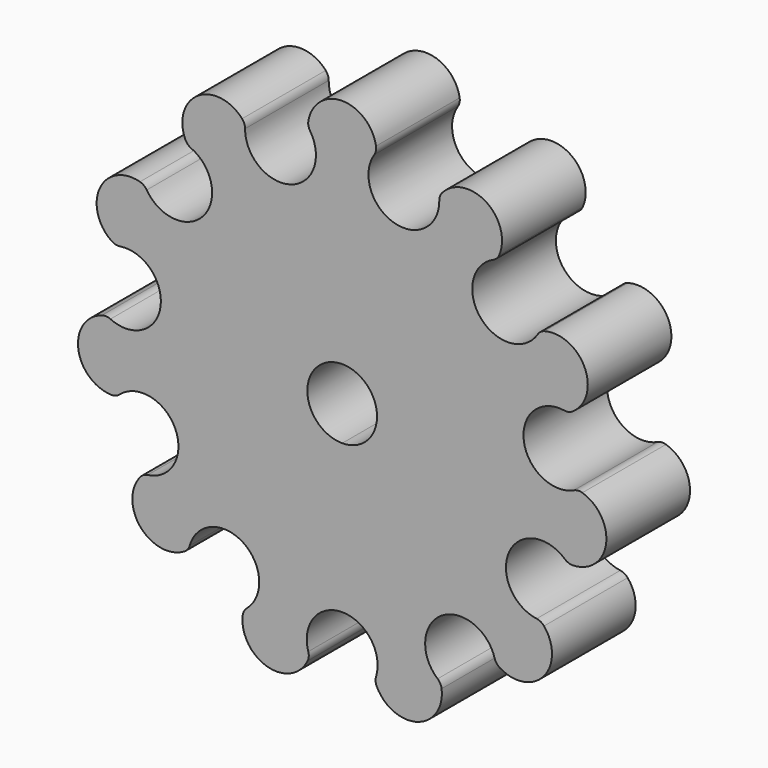
from build123d import *

# Parameters (mm, degrees)
F1_DEPTH = 9
F3_DEPTH = 25
F4_R     = 1


# Not quite as in the source:
# - a feature names something its author has since deleted; it is built from what else it names


with BuildPart() as f1:
    # F0 (on Front) → F1 (new body)
    with BuildSketch(Plane.XZ):
        with BuildLine():
            ThreePointArc((19.6162560617, 5.6676338172), (21.0365592627, 7.3533200275), (20.9215180503, 9.5545843692))
            ThreePointArc((20.9215180503, 9.5545843692), (19.3332494727, 11.0830336302), (17.1292022042, 11.1135271735))
            ThreePointArc((17.1292022042, 11.1135271735), (16.9792927626, 11.0241147009), (16.8692526077, 10.8886208073))
            ThreePointArc((16.8692526077, 10.8886208073), (14.5941945388, 9.3646392479), (12.0291450919, 10.3232477941))
            ThreePointArc((12.0291450919, 10.3232477941), (14.4190139917, 6.5849686535), (15.6791980607, 2.3307777312))
            ThreePointArc((15.6791980607, 2.3307777312), (16.6344691132, 4.8970674002), (19.2760557108, 5.6184589003))
            ThreePointArc((19.2760557108, 5.6184589003), (19.4505144763, 5.6128928995), (19.6162560617, 5.6676338172))
        make_face()
        with BuildLine():
            ThreePointArc((19.5663988928, -5.8374317411), (21.6725847499, -5.1872161444), (22.7658992762, -3.2731987637))
            ThreePointArc((22.7658992762, -3.2731987637), (22.2561047811, -1.1287026022), (20.4184282847, 0.0885481149))
            ThreePointArc((20.4184282847, 0.0885481149), (20.2439764052, 0.0943767195), (20.0781512067, 0.0398842021))
            ThreePointArc((20.0781512067, 0.0398842021), (17.3403239328, -0.0121814146), (15.7007299317, 2.1810218413))
            ThreePointArc((15.7007299317, 2.1810218413), (15.8137560479, 1.0931131305), (15.8514913071, 0))
            ThreePointArc((15.8514913071, 0), (15.497233491, -3.3324961792), (14.4502943385, -6.5160394559))
            ThreePointArc((14.4502943385, -6.5160394559), (16.6413604307, -4.8735977283), (19.2536181785, -5.6948741179))
            ThreePointArc((19.2536181785, -5.6948741179), (19.397373024, -5.7938760653), (19.5663988928, -5.8374317411))
        make_face()
        with BuildLine():
            ThreePointArc((13.4380905328, 15.3732656841), (13.7215754547, 17.5592266426), (12.4347068413, 19.3488517946))
            ThreePointArc((12.4347068413, 19.3488517946), (10.272226498, 19.7759854418), (8.4015754529, 18.610039879))
            ThreePointArc((8.4015754529, 18.610039879), (8.3238036379, 18.4537741575), (8.3044854982, 18.2802972415))
            ThreePointArc((8.3044854982, 18.2802972415), (7.2145114964, 15.7682531166), (4.5383916793, 15.1879155128))
            ThreePointArc((4.5383916793, 15.1879155128), (8.5699436247, 13.3351356547), (11.9300671826, 10.4375894572))
            ThreePointArc((11.9300671826, 10.4375894572), (11.3462513859, 13.1129482303), (13.1784817531, 15.1479709158))
            ThreePointArc((13.1784817531, 15.1479709158), (13.3282550131, 15.2376080275), (13.4380905328, 15.3732656841))
        make_face()
        with BuildLine():
            ThreePointArc((13.304348325, -15.4891539669), (15.4277177081, -16.0808478428), (17.3822683366, -15.061764421))
            ThreePointArc((17.3822683366, -15.061764421), (18.1128040767, -12.9820837356), (17.2249476546, -10.9645443445))
            ThreePointArc((17.2249476546, -10.9645443445), (17.0813405762, -10.8653252035), (16.9123786629, -10.8215153555))
            ThreePointArc((16.9123786629, -10.8215153555), (14.581022999, -9.385134564), (14.3874439542, -6.6536631357))
            ThreePointArc((14.3874439542, -6.6536631357), (11.9797730605, -10.3805016295), (8.6335242647, -13.294060156))
            ThreePointArc((8.6335242647, -13.294060156), (11.3647373936, -13.0969300134), (13.1182929141, -15.2001248417))
            ThreePointArc((13.1182929141, -15.2001248417), (13.1857026919, -15.3611303169), (13.304348325, -15.4891539669))
        make_face()
        with BuildLine():
            ThreePointArc((2.9934262088, 20.1979943186), (2.0500891812, 22.1902052175), (-3.79913e-05, 23))
            ThreePointArc((-3.79913e-05, 23), (-2.0501581038, 22.190202549), (-2.9934921419, 20.1979964151))
            ThreePointArc((-2.9934921419, 20.1979964151), (-2.9744343287, 20.0244907072), (-2.8968970802, 19.8681084639))
            ThreePointArc((-2.8968970802, 19.8681084639), (-2.4557279708, 17.1655580339), (-4.3932690247, 15.2305273689))
            ThreePointArc((-4.3932690247, 15.2305273689), (-2.32908e-05, 15.8514913071), (4.3932242679, 15.2305402791))
            ThreePointArc((4.3932242679, 15.2305402791), (2.4556790123, 17.1655606489), (2.8968329534, 19.8681091959))
            ThreePointArc((2.8968329534, 19.8681091959), (2.9743687562, 20.0244902705), (2.9934262088, 20.1979943186))
        make_face()
        with BuildLine():
            ThreePointArc((2.818261168, -20.2231792494), (4.2846548782, -21.8689217424), (6.4798805109, -22.0683290841))
            ThreePointArc((6.4798805109, -22.0683290841), (8.2188135394, -20.7137492759), (8.5626678499, -18.5364714463))
            ThreePointArc((8.5626678499, -18.5364714463), (8.4954998052, -18.3753631452), (8.3770453909, -18.2471602488))
            ThreePointArc((8.3770453909, -18.2471602488), (7.1923502876, -15.7783738016), (8.5062461781, -13.3758570797))
            ThreePointArc((8.5062461781, -13.3758570797), (4.4659035231, -15.2093879687), (0.0756712384, -15.8513106879))
            ThreePointArc((0.0756712384, -15.8513106879), (2.4798905335, -17.1620795577), (2.8180023388, -19.8794433272))
            ThreePointArc((2.8180023388, -19.8794433272), (2.7876649209, -20.0513342295), (2.818261168, -20.2231792494))
        make_face()
        with BuildLine():
            ThreePointArc((-8.4016297859, 18.6100024692), (-10.2722859221, 19.7759504243), (-12.4347707621, 19.3488107152))
            ThreePointArc((-12.4347707621, 19.3488107152), (-13.7216319934, 17.5591871352), (-13.4381471327, 15.3732318016))
            ThreePointArc((-13.4381471327, 15.3732318016), (-13.3283104123, 15.2375729436), (-13.1785353042, 15.1479356304))
            ThreePointArc((-13.1785353042, 15.1479356304), (-11.3462911586, 13.1129195615), (-11.9300978548, 10.4375543992))
            ThreePointArc((-11.9300978548, 10.4375543992), (-8.5699828116, 13.3351104708), (-4.5384363109, 15.1879021761))
            ThreePointArc((-4.5384363109, 15.1879021761), (-7.2145540967, 15.7682288475), (-8.3045398409, 18.2802631877))
            ThreePointArc((-8.3045398409, 18.2802631877), (-8.3238585649, 18.453738339), (-8.4016297859, 18.6100024692))
        make_face()
        with BuildLine():
            ThreePointArc((15.7007299317, 2.1810218413), (15.6890197856, 2.2557640279), (15.6791980607, 2.3307777312))
            ThreePointArc((15.6791980607, 2.3307777312), (14.4190139917, 6.5849686535), (12.0291450919, 10.3232477941))
            ThreePointArc((12.0291450919, 10.3232477941), (11.9788852133, 10.3797939396), (11.9300671826, 10.4375894572))
            ThreePointArc((11.9300671826, 10.4375894572), (8.5699436247, 13.3351356547), (4.5383916793, 15.1879155128))
            ThreePointArc((4.5383916793, 15.1879155128), (4.4655392245, 15.2083126157), (4.3932242679, 15.2305402791))
            ThreePointArc((4.3932242679, 15.2305402791), (-2.32908e-05, 15.8514913071), (-4.3932690247, 15.2305273689))
            ThreePointArc((-4.3932690247, 15.2305273689), (-4.4655839161, 15.2082994931), (-4.5384363109, 15.1879021761))
            ThreePointArc((-4.5384363109, 15.1879021761), (-8.5699828116, 13.3351104708), (-11.9300978548, 10.4375543992))
            ThreePointArc((-11.9300978548, 10.4375543992), (-11.9789157156, 10.3797587381), (-12.029175428, 10.3232124449))
            ThreePointArc((-12.029175428, 10.3232124449), (-14.4190333424, 6.5849262814), (-15.6792049099, 2.3307316559))
            ThreePointArc((-15.6792049099, 2.3307316559), (-15.6890264144, 2.2557179237), (-15.7007363408, 2.1809757027))
            ThreePointArc((-15.7007363408, 2.1809757027), (-15.6901426669, -2.2559254755), (-14.4502751902, -6.51608192))
            ThreePointArc((-14.4502751902, -6.51608192), (-14.41798208, -6.5844973934), (-14.3874244015, -6.6537054151))
            ThreePointArc((-14.3874244015, -6.6537054151), (-11.979742556, -10.3805368335), (-8.6334851983, -13.2940855267))
            ThreePointArc((-8.6334851983, -13.2940855267), (-8.5693303078, -13.3341813119), (-8.5062068714, -13.3758820764))
            ThreePointArc((-8.5062068714, -13.3758820764), (-4.4658588283, -15.2094010923), (-0.0756246573, -15.8513109102))
            ThreePointArc((-0.0756246573, -15.8513109102), (-0.0378153352, -15.8505955707), (0, -15.8503568788))
            ThreePointArc((0, -15.8503568788), (0.0378386269, -15.8505951659), (0.0756712384, -15.8513106879))
            ThreePointArc((0.0756712384, -15.8513106879), (4.4659035231, -15.2093879687), (8.5062461781, -13.3758570797))
            ThreePointArc((8.5062461781, -13.3758570797), (8.5693694919, -13.3341561298), (8.6335242647, -13.294060156))
            ThreePointArc((8.6335242647, -13.294060156), (11.9797730605, -10.3805016295), (14.3874439542, -6.6536631357))
            ThreePointArc((14.3874439542, -6.6536631357), (14.4180014293, -6.5844550243), (14.4502943385, -6.5160394559))
            ThreePointArc((14.4502943385, -6.5160394559), (15.497233491, -3.3324961792), (15.8514913071, 0))
            ThreePointArc((15.8514913071, 0), (15.8137560479, 1.0931131305), (15.7007299317, 2.1810218413))
        make_face()
        with BuildLine():
            ThreePointArc((2.9999669641, 0), (2.1212969837, -2.1212969837), (0, -2.9999669641))
            ThreePointArc((0, -2.9999669641), (-2.1212969837, 2.1212969837), (2.9999669641, 0))
        make_face(mode=Mode.SUBTRACT)
        with BuildLine():
            ThreePointArc((-17.1292276867, 11.1134663278), (-19.3332805342, 11.0829720434), (-20.9215496171, 9.5545152478))
            ThreePointArc((-20.9215496171, 9.5545152478), (-21.036585466, 7.3532562221), (-19.6162853583, 5.6675747132))
            ThreePointArc((-19.6162853583, 5.6675747132), (-19.4505421133, 5.612833434), (-19.2760816842, 5.6184002644))
            ThreePointArc((-19.2760816842, 5.6184002644), (-16.6344870726, 4.8970217797), (-15.6792049099, 2.3307316559))
            ThreePointArc((-15.6792049099, 2.3307316559), (-14.4190333424, 6.5849262814), (-12.029175428, 10.3232124449))
            ThreePointArc((-12.029175428, 10.3232124449), (-14.5942172556, 9.3645958), (-16.8692799128, 10.8885627796))
            ThreePointArc((-16.8692799128, 10.8885627796), (-16.9793196052, 11.0240548727), (-17.1292276867, 11.1134663278))
        make_face()
        with BuildLine():
            ThreePointArc((-8.5626039969, -18.5364880103), (-8.2187494175, -20.7137691224), (-6.4798123552, -22.0683490964))
            ThreePointArc((-6.4798123552, -22.0683490964), (-4.2845902056, -21.8689397134), (-2.8181984963, -20.2231998364))
            ThreePointArc((-2.8181984963, -20.2231998364), (-2.7876021275, -20.0513531223), (-2.8179406034, -19.8794606915))
            ThreePointArc((-2.8179406034, -19.8794606915), (-2.4798428214, -17.1620908418), (-0.0756246573, -15.8513109102))
            ThreePointArc((-0.0756246573, -15.8513109102), (-4.4658588283, -15.2094010923), (-8.5062068714, -13.3758820764))
            ThreePointArc((-8.5062068714, -13.3758820764), (-7.192304049, -15.7783901038), (-8.3769840679, -18.2471790178))
            ThreePointArc((-8.3769840679, -18.2471790178), (-8.4954367659, -18.3753812001), (-8.5626039969, -18.5364880103))
        make_face()
        with BuildLine():
            ThreePointArc((-20.4184168264, 0.0884831513), (-22.2561004524, -1.1287752683), (-22.7658870515, -3.2732837883))
            ThreePointArc((-22.7658870515, -3.2732837883), (-21.6725684309, -5.1872870865), (-19.5663915846, -5.8374973014))
            ThreePointArc((-19.5663915846, -5.8374973014), (-19.3973641243, -5.7939410325), (-19.2536083277, -5.6949374878))
            ThreePointArc((-19.2536083277, -5.6949374878), (-16.6413508748, -4.8736458164), (-14.4502751902, -6.51608192))
            ThreePointArc((-14.4502751902, -6.51608192), (-15.6901426669, -2.2559254755), (-15.7007363408, 2.1809757027))
            ThreePointArc((-15.7007363408, 2.1809757027), (-17.3403195536, -0.0122302469), (-20.078142805, 0.0398206238))
            ThreePointArc((-20.078142805, 0.0398206238), (-20.243966641, 0.0943118766), (-20.4184168264, 0.0884831513))
        make_face()
        with BuildLine():
            ThreePointArc((-17.2249028932, -10.9645928005), (-18.1127609588, -12.9821375738), (-17.3822185754, -15.0618218486))
            ThreePointArc((-17.3822185754, -15.0618218486), (-15.4276705542, -16.0808981838), (-13.3043067324, -15.4892051687))
            ThreePointArc((-13.3043067324, -15.4892051687), (-13.1856600811, -15.3611801593), (-13.1182503667, -15.2001728261))
            ThreePointArc((-13.1182503667, -15.2001728261), (-11.3647033563, -13.0969653013), (-8.6334851983, -13.2940855267))
            ThreePointArc((-8.6334851983, -13.2940855267), (-11.979742556, -10.3805368335), (-14.3874244015, -6.6537054151))
            ThreePointArc((-14.3874244015, -6.6537054151), (-14.5809929143, -9.3851732768), (-16.912337222, -10.8215642986))
            ThreePointArc((-16.912337222, -10.8215642986), (-17.0812973053, -10.865374474), (-17.2249028932, -10.9645928005))
        make_face()
    extrude(amount=F1_DEPTH)

    # F2 (on face) → F3 (cut)
    with BuildSketch(Plane(origin=(0, 0, 0), x_dir=(-1, 0, 0), z_dir=(0, 1, 0))):
        with BuildLine():
            ThreePointArc((-2.9934262088, 20.1979943186), (-2.9743687562, 20.0244902705), (-2.8968329534, 19.8681091959))
            ThreePointArc((-2.8968329534, 19.8681091959), (-4.4655438637, 15.2083112535), (-8.3044854982, 18.2802972415))
            ThreePointArc((-8.3044854982, 18.2802972415), (-8.3238036379, 18.4537741575), (-8.4015754529, 18.610039879))
            ThreePointArc((-8.4015754529, 18.610039879), (-12.4347118937, 19.3488485477), (-13.4380905328, 15.3732656841))
            ThreePointArc((-13.4380905328, 15.3732656841), (-13.3282550131, 15.2376080275), (-13.1784817531, 15.1479709158))
            ThreePointArc((-13.1784817531, 15.1479709158), (-11.9788883795, 10.3797902856), (-16.8692526077, 10.8886208073))
            ThreePointArc((-16.8692526077, 10.8886208073), (-16.9792927626, 11.0241147009), (-17.1292022042, 11.1135271735))
            ThreePointArc((-17.1292022042, 11.1135271735), (-20.9215226059, 9.5545743939), (-19.6162560617, 5.6676338172))
            ThreePointArc((-19.6162560617, 5.6676338172), (-19.4505144763, 5.6128928995), (-19.2760557108, 5.6184589003))
            ThreePointArc((-19.2760557108, 5.6184589003), (-15.6890204737, 2.2557592421), (-20.0781512067, 0.0398842021))
            ThreePointArc((-20.0781512067, 0.0398842021), (-20.2439764052, 0.0943767195), (-20.4184282847, 0.0885481149))
            ThreePointArc((-20.4184282847, 0.0885481149), (-22.7658977152, -3.2732096205), (-19.5663988928, -5.8374317411))
            ThreePointArc((-19.5663988928, -5.8374317411), (-19.397373024, -5.7938760653), (-19.2536181785, -5.6948741179))
            ThreePointArc((-19.2536181785, -5.6948741179), (-14.4179994208, -6.5844594224), (-16.9123786629, -10.8215153555))
            ThreePointArc((-16.9123786629, -10.8215153555), (-17.0813405762, -10.8653252035), (-17.2249476546, -10.9645443445))
            ThreePointArc((-17.2249476546, -10.9645443445), (-17.3822611561, -15.0617727078), (-13.304348325, -15.4891539669))
            ThreePointArc((-13.304348325, -15.4891539669), (-13.1857026919, -15.3611303169), (-13.1182929141, -15.2001248417))
            ThreePointArc((-13.1182929141, -15.2001248417), (-8.5693654245, -13.3341587438), (-8.3770453909, -18.2471602488))
            ThreePointArc((-8.3770453909, -18.2471602488), (-8.4954998052, -18.3753631452), (-8.5626678499, -18.5364714463))
            ThreePointArc((-8.5626678499, -18.5364714463), (-6.4798794971, -22.0683293818), (-2.818261168, -20.2231792494))
            ThreePointArc((-2.818261168, -20.2231792494), (-2.7876649209, -20.0513342295), (-2.8180023388, -19.8794433272))
            ThreePointArc((-2.8180023388, -19.8794433272), (-1.84541e-05, -15.8503568787), (2.8179406034, -19.8794606915))
            ThreePointArc((2.8179406034, -19.8794606915), (2.7876021275, -20.0513531223), (2.8181984963, -20.2231998364))
            ThreePointArc((2.8181984963, -20.2231998364), (6.4798181176, -22.0683474044), (8.5626039969, -18.5364880103))
            ThreePointArc((8.5626039969, -18.5364880103), (8.4954367659, -18.3753812001), (8.3769840679, -18.2471790178))
            ThreePointArc((8.3769840679, -18.2471790178), (8.5693343752, -13.3341786979), (13.1182503667, -15.2001728261))
            ThreePointArc((13.1182503667, -15.2001728261), (13.1856600811, -15.3611801593), (13.3043067324, -15.4892051687))
            ThreePointArc((13.3043067324, -15.4892051687), (17.3822192642, -15.0618210537), (17.2249028932, -10.9645928005))
            ThreePointArc((17.2249028932, -10.9645928005), (17.0812973053, -10.865374474), (16.912337222, -10.8215642986))
            ThreePointArc((16.912337222, -10.8215642986), (14.4179840885, -6.5844929953), (19.2536083277, -5.6949374878))
            ThreePointArc((19.2536083277, -5.6949374878), (19.3973641243, -5.7939410325), (19.5663915846, -5.8374973014))
            ThreePointArc((19.5663915846, -5.8374973014), (22.7658886112, -3.2732729401), (20.4184168264, 0.0884831513))
            ThreePointArc((20.4184168264, 0.0884831513), (20.243966641, 0.0943118766), (20.078142805, 0.0398206238))
            ThreePointArc((20.078142805, 0.0398206238), (15.6890257263, 2.2557227095), (19.2760816842, 5.6184002644))
            ThreePointArc((19.2760816842, 5.6184002644), (19.4505421133, 5.612833434), (19.6162853583, 5.6675747132))
            ThreePointArc((19.6162853583, 5.6675747132), (20.9215491803, 9.5545162041), (17.1292276867, 11.1134663278))
            ThreePointArc((17.1292276867, 11.1134663278), (16.9793196052, 11.0240548727), (16.8692799128, 10.8885627796))
            ThreePointArc((16.8692799128, 10.8885627796), (11.9789125493, 10.3797623922), (13.1785353042, 15.1479356304))
            ThreePointArc((13.1785353042, 15.1479356304), (13.3283104123, 15.2375729436), (13.4381471327, 15.3732318016))
            ThreePointArc((13.4381471327, 15.3732318016), (12.4347657093, 19.3488139625), (8.4016297859, 18.6100024692))
            ThreePointArc((8.4016297859, 18.6100024692), (8.3238585649, 18.453738339), (8.3045398409, 18.2802631877))
            ThreePointArc((8.3045398409, 18.2802631877), (4.4655792769, 15.2083008553), (2.8968970802, 19.8681084639))
            ThreePointArc((2.8968970802, 19.8681084639), (2.9744343287, 20.0244907072), (2.9934921419, 20.1979964151))
            ThreePointArc((2.9934921419, 20.1979964151), (3.19854e-05, 23), (-2.9934262088, 20.1979943186))
        make_face()
        with BuildLine():
            ThreePointArc((-8.340793387, 18.4349766737), (-4.4514581573, 15.1603363343), (-2.9499128846, 20.0178624202))
            ThreePointArc((-2.9499128846, 20.0178624202), (3.29413e-05, 22.95), (2.9499789552, 20.0178626094))
            ThreePointArc((2.9499789552, 20.0178626094), (4.4514917276, 15.1603264772), (8.3408488669, 18.4349407941))
            ThreePointArc((8.3408488669, 18.4349407941), (12.4077344726, 19.306750769), (13.3041538227, 15.245218606))
            ThreePointArc((13.3041538227, 15.245218606), (11.9411244417, 10.3470200813), (16.9834500367, 10.9990557209))
            ThreePointArc((16.9834500367, 10.9990557209), (20.8760679777, 9.5337445839), (19.4343538542, 5.6323254128))
            ThreePointArc((19.4343538542, 5.6323254128), (15.6395345175, 2.2486079181), (20.2339258193, 0.071048172))
            ThreePointArc((20.2339258193, 0.071048172), (22.7163974031, -3.2661581444), (19.3942838535, -5.7687913028))
            ThreePointArc((19.3942838535, -5.7687913028), (14.3725028877, -6.5637213711), (17.0602731203, -10.8795166696))
            ThreePointArc((17.0602731203, -10.8795166696), (17.3444311595, -15.0290787394), (13.1966657628, -15.3383575402))
            ThreePointArc((13.1966657628, -15.3383575402), (8.5423031423, -13.292115502), (8.4701042477, -18.3759118395))
            ThreePointArc((8.4701042477, -18.3759118395), (6.4657305726, -22.0203730251), (2.8091995356, -20.0381036342))
            ThreePointArc((2.8091995356, -20.0381036342), (-1.74938e-05, -15.8003568787), (-2.8092628766, -20.0380848384))
            ThreePointArc((-2.8092628766, -20.0380848384), (-6.4657937864, -22.0203544638), (-8.4701676953, -18.3758934068))
            ThreePointArc((-8.4701676953, -18.3758934068), (-8.5423325757, -13.2920965864), (-13.1967088869, -15.3383074835))
            ThreePointArc((-13.1967088869, -15.3383074835), (-17.3444743034, -15.0290289487), (-17.0603165303, -10.8794668606))
            ThreePointArc((-17.0603165303, -10.8794668606), (-14.3725174221, -6.5636895453), (-19.3942930691, -5.7687258778))
            ThreePointArc((-19.3942930691, -5.7687258778), (-22.7164067792, -3.2660929324), (-20.2339354093, 0.0711135432))
            ThreePointArc((-20.2339354093, 0.0711135432), (-15.6395295383, 2.2486425496), (-19.4343262354, 5.6323854342))
            ThreePointArc((-19.4343262354, 5.6323854342), (-20.8760406091, 9.5338045128), (-16.9834227621, 10.9991158995))
            ThreePointArc((-16.9834227621, 10.9991158995), (-11.9411015297, 10.3470465231), (-13.3040981383, 15.2452541674))
            ThreePointArc((-13.3040981383, 15.2452541674), (-12.4076790486, 19.3067863879), (-8.340793387, 18.4349766737))
        make_face(mode=Mode.SUBTRACT)
    extrude(amount=-F3_DEPTH, mode=Mode.SUBTRACT)

    # F4
    f4_edges = [f1.edges().sort_by_distance(p)[0] for p in [
        (19.434326, -4.5, 5.632385),
        (19.394293, -4.5, -5.768726),
        (13.304098, -4.5, 15.245254),
        (13.196709, -4.5, -15.338307),
        (-13.196666, -4.5, -15.338358),
        (-19.394284, -4.5, -5.768791),
        (-19.434354, -4.5, 5.632325),
        (-13.304154, -4.5, 15.245219),
        (2.949913, -4.5, 20.017862),
        (-8.340849, -4.5, 18.434941),
        (8.470168, -4.5, -18.375893),
        (-2.8092, -4.5, -20.038104),
        (-20.233926, -4.5, 0.071048),
        (-16.98345, -4.5, 10.999056),
        (17.060317, -4.5, -10.879467),
        (20.233935, -4.5, 0.071114),
        (16.983423, -4.5, 10.999116),
        (8.340793, -4.5, 18.434977),
        (-2.949979, -4.5, 20.017863),
        (2.809263, -4.5, -20.038085),
        (-8.470104, -4.5, -18.375912),
        (-17.060273, -4.5, -10.879517),
    ]]
    fillet(f4_edges, radius=F4_R)


solid = f1.part
